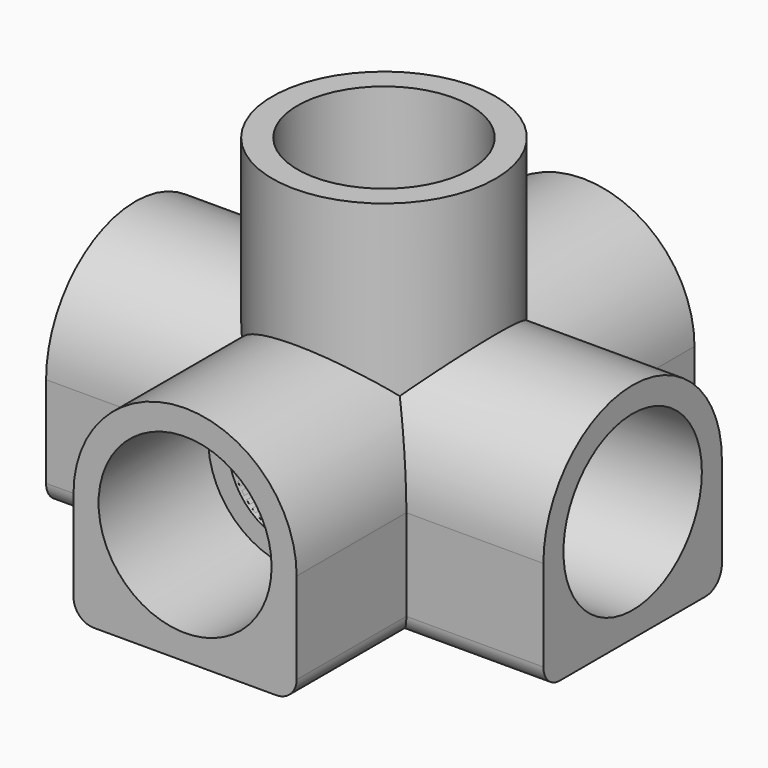
from build123d import *

# Parameters (mm, degrees)
F1_DEPTH       = 30.95625
F1_DEPTH_BACK  = 30.95625
F3_DEPTH       = 30.95625
F3_DEPTH_BACK  = 30.95625
F4_R           = 13.890625
F5_DEPTH       = 30.95625
F6_R           = 10.7696
F7_DEPTH       = 17.4625
F11_R          = 10.7696
F12_DEPTH      = 17.4625
F10_R          = 10.7696
F13_DEPTH      = 17.4625
F9_R           = 10.7696
F14_DEPTH      = 17.4625
F8_R           = 10.7696
F15_DEPTH      = 17.4625
F16_R          = 8.255
F17_DEPTH      = 61.9135
F18_R          = 8.255
F19_DEPTH      = 61.9135001
F21_END_RADIUS = 8.255
F20_R          = 8.255
F21_REACH      = 68.1965409148


with BuildPart() as f1:
    # F0 (on Front) → F1 (new body, two sides)
    with BuildSketch(Plane.XZ) as f1_sk:
        with BuildLine():
            Line((13.890625, -11.350625), (13.890625, 0))
            ThreePointArc((13.890625, 0), (0, 13.890625), (-13.890625, 0))
            Line((-13.890625, 0), (-13.890625, -11.350625))
            ThreePointArc((-13.890625, -11.350625), (-13.1466762242, -13.1466762242), (-11.350625, -13.890625))
            Line((-11.350625, -13.890625), (11.350625, -13.890625))
            ThreePointArc((11.350625, -13.890625), (13.1466762242, -13.1466762242), (13.890625, -11.350625))
        make_face()
    extrude(amount=F1_DEPTH)
    extrude(f1_sk.sketch, amount=-F1_DEPTH_BACK)

    # F6 (on face) → F7 (cut)
    with BuildSketch(Plane(origin=(0, 30.95625, 0), x_dir=(-1, 0, 0), z_dir=(0, 1, 0))):
        Circle(F6_R)
    extrude(amount=-F7_DEPTH, mode=Mode.SUBTRACT)

    # F9 (on face) → F14 (cut)
    with BuildSketch(Plane.XZ.offset(30.95625)):
        Circle(F9_R)
    extrude(amount=-F14_DEPTH, mode=Mode.SUBTRACT)


with BuildPart() as f3:
    # F2 (on Right) → F3 (new body, two sides)
    with BuildSketch(Plane.YZ) as f3_sk:
        with BuildLine():
            Line((13.890625, -11.350625), (13.890625, 0))
            ThreePointArc((13.890625, 0), (0, 13.890625), (-13.890625, 0))
            Line((-13.890625, 0), (-13.890625, -11.350625))
            ThreePointArc((-13.890625, -11.350625), (-13.1466762242, -13.1466762242), (-11.350625, -13.890625))
            Line((-11.350625, -13.890625), (11.350625, -13.890625))
            ThreePointArc((11.350625, -13.890625), (13.1466762242, -13.1466762242), (13.890625, -11.350625))
        make_face()
    extrude(amount=F3_DEPTH)
    extrude(f3_sk.sketch, amount=-F3_DEPTH_BACK)

    # F11 (on face) → F12 (cut)
    with BuildSketch(Plane.YZ.offset(30.95625)):
        Circle(F11_R)
    extrude(amount=-F12_DEPTH, mode=Mode.SUBTRACT)

    # F8 (on face) → F15 (cut)
    with BuildSketch(Plane(origin=(-30.95625, 0, 0), x_dir=(0, -1, 0), z_dir=(-1, 0, 0))):
        Circle(F8_R)
    extrude(amount=-F15_DEPTH, mode=Mode.SUBTRACT)


with BuildPart() as f5:
    # F4 (on Top) → F5 (new body)
    with BuildSketch(Plane.XY):
        Circle(F4_R)
    extrude(amount=F5_DEPTH)

    # F10 (on face) → F13 (cut)
    with BuildSketch(Plane.XY.offset(30.95625)):
        Circle(F10_R)
    extrude(amount=-F13_DEPTH, mode=Mode.SUBTRACT)


with BuildPart() as f17_tool:
    # F16 (on face) → F17 (new body, through all)
    with BuildSketch(Plane.XZ.offset(30.95625)):
        Circle(F16_R)
    extrude(amount=-F17_DEPTH)


with BuildPart() as f1_1:
    add(f1.part)

    # F17: cut by f17_tool
    add(f17_tool.part, mode=Mode.SUBTRACT)


with BuildPart() as f3_1:
    add(f3.part)

    # F17: cut by f17_tool
    add(f17_tool.part, mode=Mode.SUBTRACT)


with BuildPart() as f5_1:
    add(f5.part)

    # F17: cut by f17_tool
    add(f17_tool.part, mode=Mode.SUBTRACT)


with BuildPart() as f19_tool:
    # F18 (on face) → F19 (new body, through all)
    with BuildSketch(Plane.YZ.offset(30.95625)):
        Circle(F18_R)
    extrude(amount=-F19_DEPTH)


with BuildPart() as f1_2:
    add(f1_1.part)

    # F19: cut by f19_tool
    add(f19_tool.part, mode=Mode.SUBTRACT)


with BuildPart() as f3_2:
    add(f3_1.part)

    # F19: cut by f19_tool
    add(f19_tool.part, mode=Mode.SUBTRACT)


with BuildPart() as f5_2:
    add(f5_1.part)

    # F19: cut by f19_tool
    add(f19_tool.part, mode=Mode.SUBTRACT)


with BuildPart() as f21_tool:
    f21_end = (Plane(origin=(-6.9453125, 0, 0), x_dir=(0, 0, 1), z_dir=(1, 0, 0)) * Cylinder(F21_END_RADIUS, 333.1422375407, mode=Mode.PRIVATE)).faces().sort_by_distance((-13.6189432594, 0, -8.255))[0]
    # F20 (on face) → F21 (new body, up to the whole of a round face its end follows)
    with BuildSketch(Plane.XY.offset(30.95625)):
        Circle(F20_R)
    f21_long = extrude(amount=-F21_REACH, mode=Mode.PRIVATE)
    add(split(f21_long, bisect_by=f21_end, keep=Keep.ALL, mode=Mode.PRIVATE).solids().sort_by_distance((0, 0, 30.95625))[0])


with BuildPart() as f1_3:
    add(f1_2.part)

    # F21: cut by f21_tool
    add(f21_tool.part, mode=Mode.SUBTRACT)


with BuildPart() as f3_3:
    add(f3_2.part)

    # F21: cut by f21_tool
    add(f21_tool.part, mode=Mode.SUBTRACT)


with BuildPart() as f5_3:
    add(f5_2.part)

    # F21: cut by f21_tool
    add(f21_tool.part, mode=Mode.SUBTRACT)


solid = Compound([f1_3.part, f3_3.part, f5_3.part])
